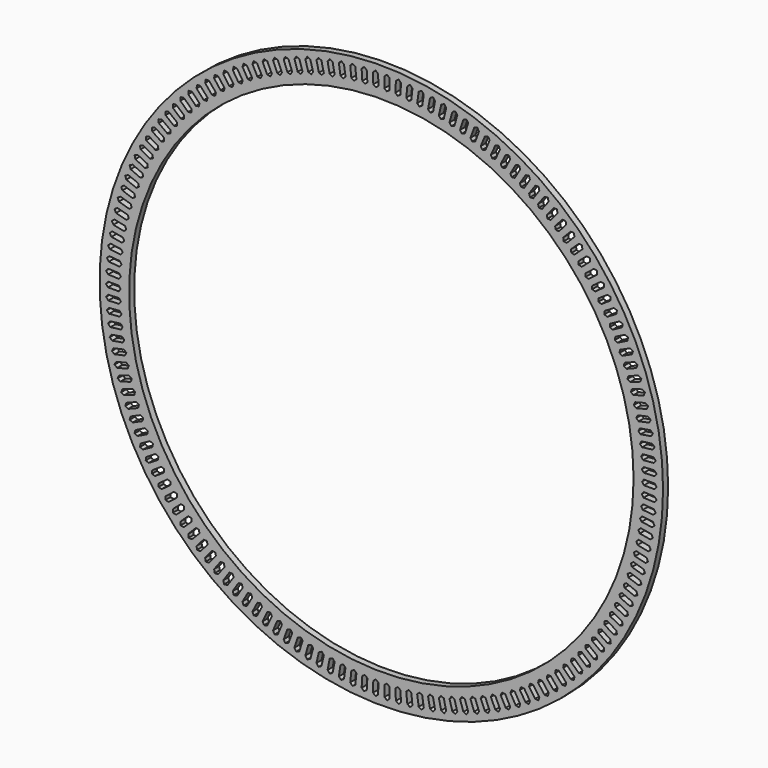
from build123d import *

# Parameters (mm, degrees)
F0_R     = 44.4451072214
F0_R_2   = 39.7909851914
F1_DEPTH = 1
F3_DEPTH = 1
F4_COUNT = 150
F6_SCALE = 2.61


with BuildPart() as f1:
    # F0 (on Front) → F1 (new body)
    with BuildSketch(Plane.XZ):
        Circle(F0_R)
        Circle(F0_R_2, mode=Mode.SUBTRACT)
    extrude(amount=-F1_DEPTH)


with BuildPart() as f3:
    # F2 (on Front) → F3 (new body)
    with BuildSketch(Plane.XZ):
        Polygon((-41.4202045649, 0.4029835982), (-43.1122351438, 0.4029835982), (-43.4538759291, 0), (-43.1122351438, -0.4029835982), (-41.4202045649, -0.4029835982), (-41.1230549216, 0), align=None)
    extrude(amount=-F3_DEPTH)


with BuildPart() as f4_1:
    # F4: instance of F3
    add(f3.part.rotate(Axis((0, 0, 0), (0, -1, 0)), 1 * 360 / F4_COUNT))


with BuildPart() as f4_2:
    # F4: instance of F3
    add(f3.part.rotate(Axis((0, 0, 0), (0, -1, 0)), 2 * 360 / F4_COUNT))


with BuildPart() as f4_3:
    # F4: instance of F3
    add(f3.part.rotate(Axis((0, 0, 0), (0, -1, 0)), 3 * 360 / F4_COUNT))


with BuildPart() as f4_4:
    # F4: instance of F3
    add(f3.part.rotate(Axis((0, 0, 0), (0, -1, 0)), 4 * 360 / F4_COUNT))


with BuildPart() as f4_5:
    # F4: instance of F3
    add(f3.part.rotate(Axis((0, 0, 0), (0, -1, 0)), 5 * 360 / F4_COUNT))


with BuildPart() as f4_6:
    # F4: instance of F3
    add(f3.part.rotate(Axis((0, 0, 0), (0, -1, 0)), 6 * 360 / F4_COUNT))


with BuildPart() as f4_7:
    # F4: instance of F3
    add(f3.part.rotate(Axis((0, 0, 0), (0, -1, 0)), 7 * 360 / F4_COUNT))


with BuildPart() as f4_8:
    # F4: instance of F3
    add(f3.part.rotate(Axis((0, 0, 0), (0, -1, 0)), 8 * 360 / F4_COUNT))


with BuildPart() as f4_9:
    # F4: instance of F3
    add(f3.part.rotate(Axis((0, 0, 0), (0, -1, 0)), 9 * 360 / F4_COUNT))


with BuildPart() as f4_10:
    # F4: instance of F3
    add(f3.part.rotate(Axis((0, 0, 0), (0, -1, 0)), 10 * 360 / F4_COUNT))


with BuildPart() as f4_11:
    # F4: instance of F3
    add(f3.part.rotate(Axis((0, 0, 0), (0, -1, 0)), 11 * 360 / F4_COUNT))


with BuildPart() as f4_12:
    # F4: instance of F3
    add(f3.part.rotate(Axis((0, 0, 0), (0, -1, 0)), 12 * 360 / F4_COUNT))


with BuildPart() as f4_13:
    # F4: instance of F3
    add(f3.part.rotate(Axis((0, 0, 0), (0, -1, 0)), 13 * 360 / F4_COUNT))


with BuildPart() as f4_14:
    # F4: instance of F3
    add(f3.part.rotate(Axis((0, 0, 0), (0, -1, 0)), 14 * 360 / F4_COUNT))


with BuildPart() as f4_15:
    # F4: instance of F3
    add(f3.part.rotate(Axis((0, 0, 0), (0, -1, 0)), 15 * 360 / F4_COUNT))


with BuildPart() as f4_16:
    # F4: instance of F3
    add(f3.part.rotate(Axis((0, 0, 0), (0, -1, 0)), 16 * 360 / F4_COUNT))


with BuildPart() as f4_17:
    # F4: instance of F3
    add(f3.part.rotate(Axis((0, 0, 0), (0, -1, 0)), 17 * 360 / F4_COUNT))


with BuildPart() as f4_18:
    # F4: instance of F3
    add(f3.part.rotate(Axis((0, 0, 0), (0, -1, 0)), 18 * 360 / F4_COUNT))


with BuildPart() as f4_19:
    # F4: instance of F3
    add(f3.part.rotate(Axis((0, 0, 0), (0, -1, 0)), 19 * 360 / F4_COUNT))


with BuildPart() as f4_20:
    # F4: instance of F3
    add(f3.part.rotate(Axis((0, 0, 0), (0, -1, 0)), 20 * 360 / F4_COUNT))


with BuildPart() as f4_21:
    # F4: instance of F3
    add(f3.part.rotate(Axis((0, 0, 0), (0, -1, 0)), 21 * 360 / F4_COUNT))


with BuildPart() as f4_22:
    # F4: instance of F3
    add(f3.part.rotate(Axis((0, 0, 0), (0, -1, 0)), 22 * 360 / F4_COUNT))


with BuildPart() as f4_23:
    # F4: instance of F3
    add(f3.part.rotate(Axis((0, 0, 0), (0, -1, 0)), 23 * 360 / F4_COUNT))


with BuildPart() as f4_24:
    # F4: instance of F3
    add(f3.part.rotate(Axis((0, 0, 0), (0, -1, 0)), 24 * 360 / F4_COUNT))


with BuildPart() as f4_25:
    # F4: instance of F3
    add(f3.part.rotate(Axis((0, 0, 0), (0, -1, 0)), 25 * 360 / F4_COUNT))


with BuildPart() as f4_26:
    # F4: instance of F3
    add(f3.part.rotate(Axis((0, 0, 0), (0, -1, 0)), 26 * 360 / F4_COUNT))


with BuildPart() as f4_27:
    # F4: instance of F3
    add(f3.part.rotate(Axis((0, 0, 0), (0, -1, 0)), 27 * 360 / F4_COUNT))


with BuildPart() as f4_28:
    # F4: instance of F3
    add(f3.part.rotate(Axis((0, 0, 0), (0, -1, 0)), 28 * 360 / F4_COUNT))


with BuildPart() as f4_29:
    # F4: instance of F3
    add(f3.part.rotate(Axis((0, 0, 0), (0, -1, 0)), 29 * 360 / F4_COUNT))


with BuildPart() as f4_30:
    # F4: instance of F3
    add(f3.part.rotate(Axis((0, 0, 0), (0, -1, 0)), 30 * 360 / F4_COUNT))


with BuildPart() as f4_31:
    # F4: instance of F3
    add(f3.part.rotate(Axis((0, 0, 0), (0, -1, 0)), 31 * 360 / F4_COUNT))


with BuildPart() as f4_32:
    # F4: instance of F3
    add(f3.part.rotate(Axis((0, 0, 0), (0, -1, 0)), 32 * 360 / F4_COUNT))


with BuildPart() as f4_33:
    # F4: instance of F3
    add(f3.part.rotate(Axis((0, 0, 0), (0, -1, 0)), 33 * 360 / F4_COUNT))


with BuildPart() as f4_34:
    # F4: instance of F3
    add(f3.part.rotate(Axis((0, 0, 0), (0, -1, 0)), 34 * 360 / F4_COUNT))


with BuildPart() as f4_35:
    # F4: instance of F3
    add(f3.part.rotate(Axis((0, 0, 0), (0, -1, 0)), 35 * 360 / F4_COUNT))


with BuildPart() as f4_36:
    # F4: instance of F3
    add(f3.part.rotate(Axis((0, 0, 0), (0, -1, 0)), 36 * 360 / F4_COUNT))


with BuildPart() as f4_37:
    # F4: instance of F3
    add(f3.part.rotate(Axis((0, 0, 0), (0, -1, 0)), 37 * 360 / F4_COUNT))


with BuildPart() as f4_38:
    # F4: instance of F3
    add(f3.part.rotate(Axis((0, 0, 0), (0, -1, 0)), 38 * 360 / F4_COUNT))


with BuildPart() as f4_39:
    # F4: instance of F3
    add(f3.part.rotate(Axis((0, 0, 0), (0, -1, 0)), 39 * 360 / F4_COUNT))


with BuildPart() as f4_40:
    # F4: instance of F3
    add(f3.part.rotate(Axis((0, 0, 0), (0, -1, 0)), 40 * 360 / F4_COUNT))


with BuildPart() as f4_41:
    # F4: instance of F3
    add(f3.part.rotate(Axis((0, 0, 0), (0, -1, 0)), 41 * 360 / F4_COUNT))


with BuildPart() as f4_42:
    # F4: instance of F3
    add(f3.part.rotate(Axis((0, 0, 0), (0, -1, 0)), 42 * 360 / F4_COUNT))


with BuildPart() as f4_43:
    # F4: instance of F3
    add(f3.part.rotate(Axis((0, 0, 0), (0, -1, 0)), 43 * 360 / F4_COUNT))


with BuildPart() as f4_44:
    # F4: instance of F3
    add(f3.part.rotate(Axis((0, 0, 0), (0, -1, 0)), 44 * 360 / F4_COUNT))


with BuildPart() as f4_45:
    # F4: instance of F3
    add(f3.part.rotate(Axis((0, 0, 0), (0, -1, 0)), 45 * 360 / F4_COUNT))


with BuildPart() as f4_46:
    # F4: instance of F3
    add(f3.part.rotate(Axis((0, 0, 0), (0, -1, 0)), 46 * 360 / F4_COUNT))


with BuildPart() as f4_47:
    # F4: instance of F3
    add(f3.part.rotate(Axis((0, 0, 0), (0, -1, 0)), 47 * 360 / F4_COUNT))


with BuildPart() as f4_48:
    # F4: instance of F3
    add(f3.part.rotate(Axis((0, 0, 0), (0, -1, 0)), 48 * 360 / F4_COUNT))


with BuildPart() as f4_49:
    # F4: instance of F3
    add(f3.part.rotate(Axis((0, 0, 0), (0, -1, 0)), 49 * 360 / F4_COUNT))


with BuildPart() as f4_50:
    # F4: instance of F3
    add(f3.part.rotate(Axis((0, 0, 0), (0, -1, 0)), 50 * 360 / F4_COUNT))


with BuildPart() as f4_51:
    # F4: instance of F3
    add(f3.part.rotate(Axis((0, 0, 0), (0, -1, 0)), 51 * 360 / F4_COUNT))


with BuildPart() as f4_52:
    # F4: instance of F3
    add(f3.part.rotate(Axis((0, 0, 0), (0, -1, 0)), 52 * 360 / F4_COUNT))


with BuildPart() as f4_53:
    # F4: instance of F3
    add(f3.part.rotate(Axis((0, 0, 0), (0, -1, 0)), 53 * 360 / F4_COUNT))


with BuildPart() as f4_54:
    # F4: instance of F3
    add(f3.part.rotate(Axis((0, 0, 0), (0, -1, 0)), 54 * 360 / F4_COUNT))


with BuildPart() as f4_55:
    # F4: instance of F3
    add(f3.part.rotate(Axis((0, 0, 0), (0, -1, 0)), 55 * 360 / F4_COUNT))


with BuildPart() as f4_56:
    # F4: instance of F3
    add(f3.part.rotate(Axis((0, 0, 0), (0, -1, 0)), 56 * 360 / F4_COUNT))


with BuildPart() as f4_57:
    # F4: instance of F3
    add(f3.part.rotate(Axis((0, 0, 0), (0, -1, 0)), 57 * 360 / F4_COUNT))


with BuildPart() as f4_58:
    # F4: instance of F3
    add(f3.part.rotate(Axis((0, 0, 0), (0, -1, 0)), 58 * 360 / F4_COUNT))


with BuildPart() as f4_59:
    # F4: instance of F3
    add(f3.part.rotate(Axis((0, 0, 0), (0, -1, 0)), 59 * 360 / F4_COUNT))


with BuildPart() as f4_60:
    # F4: instance of F3
    add(f3.part.rotate(Axis((0, 0, 0), (0, -1, 0)), 60 * 360 / F4_COUNT))


with BuildPart() as f4_61:
    # F4: instance of F3
    add(f3.part.rotate(Axis((0, 0, 0), (0, -1, 0)), 61 * 360 / F4_COUNT))


with BuildPart() as f4_62:
    # F4: instance of F3
    add(f3.part.rotate(Axis((0, 0, 0), (0, -1, 0)), 62 * 360 / F4_COUNT))


with BuildPart() as f4_63:
    # F4: instance of F3
    add(f3.part.rotate(Axis((0, 0, 0), (0, -1, 0)), 63 * 360 / F4_COUNT))


with BuildPart() as f4_64:
    # F4: instance of F3
    add(f3.part.rotate(Axis((0, 0, 0), (0, -1, 0)), 64 * 360 / F4_COUNT))


with BuildPart() as f4_65:
    # F4: instance of F3
    add(f3.part.rotate(Axis((0, 0, 0), (0, -1, 0)), 65 * 360 / F4_COUNT))


with BuildPart() as f4_66:
    # F4: instance of F3
    add(f3.part.rotate(Axis((0, 0, 0), (0, -1, 0)), 66 * 360 / F4_COUNT))


with BuildPart() as f4_67:
    # F4: instance of F3
    add(f3.part.rotate(Axis((0, 0, 0), (0, -1, 0)), 67 * 360 / F4_COUNT))


with BuildPart() as f4_68:
    # F4: instance of F3
    add(f3.part.rotate(Axis((0, 0, 0), (0, -1, 0)), 68 * 360 / F4_COUNT))


with BuildPart() as f4_69:
    # F4: instance of F3
    add(f3.part.rotate(Axis((0, 0, 0), (0, -1, 0)), 69 * 360 / F4_COUNT))


with BuildPart() as f4_70:
    # F4: instance of F3
    add(f3.part.rotate(Axis((0, 0, 0), (0, -1, 0)), 70 * 360 / F4_COUNT))


with BuildPart() as f4_71:
    # F4: instance of F3
    add(f3.part.rotate(Axis((0, 0, 0), (0, -1, 0)), 71 * 360 / F4_COUNT))


with BuildPart() as f4_72:
    # F4: instance of F3
    add(f3.part.rotate(Axis((0, 0, 0), (0, -1, 0)), 72 * 360 / F4_COUNT))


with BuildPart() as f4_73:
    # F4: instance of F3
    add(f3.part.rotate(Axis((0, 0, 0), (0, -1, 0)), 73 * 360 / F4_COUNT))


with BuildPart() as f4_74:
    # F4: instance of F3
    add(f3.part.rotate(Axis((0, 0, 0), (0, -1, 0)), 74 * 360 / F4_COUNT))


with BuildPart() as f4_75:
    # F4: instance of F3
    add(f3.part.rotate(Axis((0, 0, 0), (0, -1, 0)), 75 * 360 / F4_COUNT))


with BuildPart() as f4_76:
    # F4: instance of F3
    add(f3.part.rotate(Axis((0, 0, 0), (0, -1, 0)), 76 * 360 / F4_COUNT))


with BuildPart() as f4_77:
    # F4: instance of F3
    add(f3.part.rotate(Axis((0, 0, 0), (0, -1, 0)), 77 * 360 / F4_COUNT))


with BuildPart() as f4_78:
    # F4: instance of F3
    add(f3.part.rotate(Axis((0, 0, 0), (0, -1, 0)), 78 * 360 / F4_COUNT))


with BuildPart() as f4_79:
    # F4: instance of F3
    add(f3.part.rotate(Axis((0, 0, 0), (0, -1, 0)), 79 * 360 / F4_COUNT))


with BuildPart() as f4_80:
    # F4: instance of F3
    add(f3.part.rotate(Axis((0, 0, 0), (0, -1, 0)), 80 * 360 / F4_COUNT))


with BuildPart() as f4_81:
    # F4: instance of F3
    add(f3.part.rotate(Axis((0, 0, 0), (0, -1, 0)), 81 * 360 / F4_COUNT))


with BuildPart() as f4_82:
    # F4: instance of F3
    add(f3.part.rotate(Axis((0, 0, 0), (0, -1, 0)), 82 * 360 / F4_COUNT))


with BuildPart() as f4_83:
    # F4: instance of F3
    add(f3.part.rotate(Axis((0, 0, 0), (0, -1, 0)), 83 * 360 / F4_COUNT))


with BuildPart() as f4_84:
    # F4: instance of F3
    add(f3.part.rotate(Axis((0, 0, 0), (0, -1, 0)), 84 * 360 / F4_COUNT))


with BuildPart() as f4_85:
    # F4: instance of F3
    add(f3.part.rotate(Axis((0, 0, 0), (0, -1, 0)), 85 * 360 / F4_COUNT))


with BuildPart() as f4_86:
    # F4: instance of F3
    add(f3.part.rotate(Axis((0, 0, 0), (0, -1, 0)), 86 * 360 / F4_COUNT))


with BuildPart() as f4_87:
    # F4: instance of F3
    add(f3.part.rotate(Axis((0, 0, 0), (0, -1, 0)), 87 * 360 / F4_COUNT))


with BuildPart() as f4_88:
    # F4: instance of F3
    add(f3.part.rotate(Axis((0, 0, 0), (0, -1, 0)), 88 * 360 / F4_COUNT))


with BuildPart() as f4_89:
    # F4: instance of F3
    add(f3.part.rotate(Axis((0, 0, 0), (0, -1, 0)), 89 * 360 / F4_COUNT))


with BuildPart() as f4_90:
    # F4: instance of F3
    add(f3.part.rotate(Axis((0, 0, 0), (0, -1, 0)), 90 * 360 / F4_COUNT))


with BuildPart() as f4_91:
    # F4: instance of F3
    add(f3.part.rotate(Axis((0, 0, 0), (0, -1, 0)), 91 * 360 / F4_COUNT))


with BuildPart() as f4_92:
    # F4: instance of F3
    add(f3.part.rotate(Axis((0, 0, 0), (0, -1, 0)), 92 * 360 / F4_COUNT))


with BuildPart() as f4_93:
    # F4: instance of F3
    add(f3.part.rotate(Axis((0, 0, 0), (0, -1, 0)), 93 * 360 / F4_COUNT))


with BuildPart() as f4_94:
    # F4: instance of F3
    add(f3.part.rotate(Axis((0, 0, 0), (0, -1, 0)), 94 * 360 / F4_COUNT))


with BuildPart() as f4_95:
    # F4: instance of F3
    add(f3.part.rotate(Axis((0, 0, 0), (0, -1, 0)), 95 * 360 / F4_COUNT))


with BuildPart() as f4_96:
    # F4: instance of F3
    add(f3.part.rotate(Axis((0, 0, 0), (0, -1, 0)), 96 * 360 / F4_COUNT))


with BuildPart() as f4_97:
    # F4: instance of F3
    add(f3.part.rotate(Axis((0, 0, 0), (0, -1, 0)), 97 * 360 / F4_COUNT))


with BuildPart() as f4_98:
    # F4: instance of F3
    add(f3.part.rotate(Axis((0, 0, 0), (0, -1, 0)), 98 * 360 / F4_COUNT))


with BuildPart() as f4_99:
    # F4: instance of F3
    add(f3.part.rotate(Axis((0, 0, 0), (0, -1, 0)), 99 * 360 / F4_COUNT))


with BuildPart() as f4_100:
    # F4: instance of F3
    add(f3.part.rotate(Axis((0, 0, 0), (0, -1, 0)), 100 * 360 / F4_COUNT))


with BuildPart() as f4_101:
    # F4: instance of F3
    add(f3.part.rotate(Axis((0, 0, 0), (0, -1, 0)), 101 * 360 / F4_COUNT))


with BuildPart() as f4_102:
    # F4: instance of F3
    add(f3.part.rotate(Axis((0, 0, 0), (0, -1, 0)), 102 * 360 / F4_COUNT))


with BuildPart() as f4_103:
    # F4: instance of F3
    add(f3.part.rotate(Axis((0, 0, 0), (0, -1, 0)), 103 * 360 / F4_COUNT))


with BuildPart() as f4_104:
    # F4: instance of F3
    add(f3.part.rotate(Axis((0, 0, 0), (0, -1, 0)), 104 * 360 / F4_COUNT))


with BuildPart() as f4_105:
    # F4: instance of F3
    add(f3.part.rotate(Axis((0, 0, 0), (0, -1, 0)), 105 * 360 / F4_COUNT))


with BuildPart() as f4_106:
    # F4: instance of F3
    add(f3.part.rotate(Axis((0, 0, 0), (0, -1, 0)), 106 * 360 / F4_COUNT))


with BuildPart() as f4_107:
    # F4: instance of F3
    add(f3.part.rotate(Axis((0, 0, 0), (0, -1, 0)), 107 * 360 / F4_COUNT))


with BuildPart() as f4_108:
    # F4: instance of F3
    add(f3.part.rotate(Axis((0, 0, 0), (0, -1, 0)), 108 * 360 / F4_COUNT))


with BuildPart() as f4_109:
    # F4: instance of F3
    add(f3.part.rotate(Axis((0, 0, 0), (0, -1, 0)), 109 * 360 / F4_COUNT))


with BuildPart() as f4_110:
    # F4: instance of F3
    add(f3.part.rotate(Axis((0, 0, 0), (0, -1, 0)), 110 * 360 / F4_COUNT))


with BuildPart() as f4_111:
    # F4: instance of F3
    add(f3.part.rotate(Axis((0, 0, 0), (0, -1, 0)), 111 * 360 / F4_COUNT))


with BuildPart() as f4_112:
    # F4: instance of F3
    add(f3.part.rotate(Axis((0, 0, 0), (0, -1, 0)), 112 * 360 / F4_COUNT))


with BuildPart() as f4_113:
    # F4: instance of F3
    add(f3.part.rotate(Axis((0, 0, 0), (0, -1, 0)), 113 * 360 / F4_COUNT))


with BuildPart() as f4_114:
    # F4: instance of F3
    add(f3.part.rotate(Axis((0, 0, 0), (0, -1, 0)), 114 * 360 / F4_COUNT))


with BuildPart() as f4_115:
    # F4: instance of F3
    add(f3.part.rotate(Axis((0, 0, 0), (0, -1, 0)), 115 * 360 / F4_COUNT))


with BuildPart() as f4_116:
    # F4: instance of F3
    add(f3.part.rotate(Axis((0, 0, 0), (0, -1, 0)), 116 * 360 / F4_COUNT))


with BuildPart() as f4_117:
    # F4: instance of F3
    add(f3.part.rotate(Axis((0, 0, 0), (0, -1, 0)), 117 * 360 / F4_COUNT))


with BuildPart() as f4_118:
    # F4: instance of F3
    add(f3.part.rotate(Axis((0, 0, 0), (0, -1, 0)), 118 * 360 / F4_COUNT))


with BuildPart() as f4_119:
    # F4: instance of F3
    add(f3.part.rotate(Axis((0, 0, 0), (0, -1, 0)), 119 * 360 / F4_COUNT))


with BuildPart() as f4_120:
    # F4: instance of F3
    add(f3.part.rotate(Axis((0, 0, 0), (0, -1, 0)), 120 * 360 / F4_COUNT))


with BuildPart() as f4_121:
    # F4: instance of F3
    add(f3.part.rotate(Axis((0, 0, 0), (0, -1, 0)), 121 * 360 / F4_COUNT))


with BuildPart() as f4_122:
    # F4: instance of F3
    add(f3.part.rotate(Axis((0, 0, 0), (0, -1, 0)), 122 * 360 / F4_COUNT))


with BuildPart() as f4_123:
    # F4: instance of F3
    add(f3.part.rotate(Axis((0, 0, 0), (0, -1, 0)), 123 * 360 / F4_COUNT))


with BuildPart() as f4_124:
    # F4: instance of F3
    add(f3.part.rotate(Axis((0, 0, 0), (0, -1, 0)), 124 * 360 / F4_COUNT))


with BuildPart() as f4_125:
    # F4: instance of F3
    add(f3.part.rotate(Axis((0, 0, 0), (0, -1, 0)), 125 * 360 / F4_COUNT))


with BuildPart() as f4_126:
    # F4: instance of F3
    add(f3.part.rotate(Axis((0, 0, 0), (0, -1, 0)), 126 * 360 / F4_COUNT))


with BuildPart() as f4_127:
    # F4: instance of F3
    add(f3.part.rotate(Axis((0, 0, 0), (0, -1, 0)), 127 * 360 / F4_COUNT))


with BuildPart() as f4_128:
    # F4: instance of F3
    add(f3.part.rotate(Axis((0, 0, 0), (0, -1, 0)), 128 * 360 / F4_COUNT))


with BuildPart() as f4_129:
    # F4: instance of F3
    add(f3.part.rotate(Axis((0, 0, 0), (0, -1, 0)), 129 * 360 / F4_COUNT))


with BuildPart() as f4_130:
    # F4: instance of F3
    add(f3.part.rotate(Axis((0, 0, 0), (0, -1, 0)), 130 * 360 / F4_COUNT))


with BuildPart() as f4_131:
    # F4: instance of F3
    add(f3.part.rotate(Axis((0, 0, 0), (0, -1, 0)), 131 * 360 / F4_COUNT))


with BuildPart() as f4_132:
    # F4: instance of F3
    add(f3.part.rotate(Axis((0, 0, 0), (0, -1, 0)), 132 * 360 / F4_COUNT))


with BuildPart() as f4_133:
    # F4: instance of F3
    add(f3.part.rotate(Axis((0, 0, 0), (0, -1, 0)), 133 * 360 / F4_COUNT))


with BuildPart() as f4_134:
    # F4: instance of F3
    add(f3.part.rotate(Axis((0, 0, 0), (0, -1, 0)), 134 * 360 / F4_COUNT))


with BuildPart() as f4_135:
    # F4: instance of F3
    add(f3.part.rotate(Axis((0, 0, 0), (0, -1, 0)), 135 * 360 / F4_COUNT))


with BuildPart() as f4_136:
    # F4: instance of F3
    add(f3.part.rotate(Axis((0, 0, 0), (0, -1, 0)), 136 * 360 / F4_COUNT))


with BuildPart() as f4_137:
    # F4: instance of F3
    add(f3.part.rotate(Axis((0, 0, 0), (0, -1, 0)), 137 * 360 / F4_COUNT))


with BuildPart() as f4_138:
    # F4: instance of F3
    add(f3.part.rotate(Axis((0, 0, 0), (0, -1, 0)), 138 * 360 / F4_COUNT))


with BuildPart() as f4_139:
    # F4: instance of F3
    add(f3.part.rotate(Axis((0, 0, 0), (0, -1, 0)), 139 * 360 / F4_COUNT))


with BuildPart() as f4_140:
    # F4: instance of F3
    add(f3.part.rotate(Axis((0, 0, 0), (0, -1, 0)), 140 * 360 / F4_COUNT))


with BuildPart() as f4_141:
    # F4: instance of F3
    add(f3.part.rotate(Axis((0, 0, 0), (0, -1, 0)), 141 * 360 / F4_COUNT))


with BuildPart() as f4_142:
    # F4: instance of F3
    add(f3.part.rotate(Axis((0, 0, 0), (0, -1, 0)), 142 * 360 / F4_COUNT))


with BuildPart() as f4_143:
    # F4: instance of F3
    add(f3.part.rotate(Axis((0, 0, 0), (0, -1, 0)), 143 * 360 / F4_COUNT))


with BuildPart() as f4_144:
    # F4: instance of F3
    add(f3.part.rotate(Axis((0, 0, 0), (0, -1, 0)), 144 * 360 / F4_COUNT))


with BuildPart() as f4_145:
    # F4: instance of F3
    add(f3.part.rotate(Axis((0, 0, 0), (0, -1, 0)), 145 * 360 / F4_COUNT))


with BuildPart() as f4_146:
    # F4: instance of F3
    add(f3.part.rotate(Axis((0, 0, 0), (0, -1, 0)), 146 * 360 / F4_COUNT))


with BuildPart() as f4_147:
    # F4: instance of F3
    add(f3.part.rotate(Axis((0, 0, 0), (0, -1, 0)), 147 * 360 / F4_COUNT))


with BuildPart() as f4_148:
    # F4: instance of F3
    add(f3.part.rotate(Axis((0, 0, 0), (0, -1, 0)), 148 * 360 / F4_COUNT))


with BuildPart() as f4_149:
    # F4: instance of F3
    add(f3.part.rotate(Axis((0, 0, 0), (0, -1, 0)), 149 * 360 / F4_COUNT))


with BuildPart() as f1_1:
    add(f1.part)

    # F5: cut F4_5, F4_6, F4_4, F4_23, F4_21, F4_24, F4_22, F4_20, F4_19, F4_18, F4_17, F4_16, F4_15, F4_14, F4_13, F4_12, F4_11, F4_10, F4_9, F4_8, F4_7, F4_1, F4_3, F4_2, F3, F4_149, F4_148, F4_147, F4_25, F4_26, F4_27, F4_28, F4_29, F4_30, F4_31, F4_32, F4_33, F4_34, F4_35, F4_36, F4_37, F4_38, F4_39, F4_40, F4_41, F4_42, F4_43, F4_44, F4_45, F4_46, F4_47, F4_48, F4_49, F4_50, F4_51, F4_52, F4_53, F4_54, F4_55, F4_56, F4_57, F4_58, F4_59, F4_60, F4_61, F4_62, F4_63, F4_64, F4_65, F4_66, F4_67, F4_68, F4_69, F4_70, F4_71, F4_72, F4_73, F4_74, F4_75, F4_76, F4_77, F4_78, F4_79, F4_80, F4_81, F4_82, F4_83, F4_84, F4_85, F4_86, F4_87, F4_88, F4_89, F4_90, F4_91, F4_92, F4_93, F4_94, F4_95, F4_96, F4_97, F4_98, F4_99, F4_100, F4_101, F4_102, F4_103, F4_104, F4_105, F4_106, F4_107, F4_108, F4_109, F4_110, F4_111, F4_112, F4_113, F4_114, F4_115, F4_116, F4_117, F4_118, F4_119, F4_120, F4_121, F4_122, F4_123, F4_124, F4_125, F4_126, F4_127, F4_128, F4_129, F4_130, F4_131, F4_132, F4_133, F4_134, F4_135, F4_136, F4_137, F4_138, F4_139, F4_140, F4_141, F4_142, F4_143, F4_144, F4_145, F4_146
    add(f4_5.part, mode=Mode.SUBTRACT)
    add(f4_6.part, mode=Mode.SUBTRACT)
    add(f4_4.part, mode=Mode.SUBTRACT)
    add(f4_23.part, mode=Mode.SUBTRACT)
    add(f4_21.part, mode=Mode.SUBTRACT)
    add(f4_24.part, mode=Mode.SUBTRACT)
    add(f4_22.part, mode=Mode.SUBTRACT)
    add(f4_20.part, mode=Mode.SUBTRACT)
    add(f4_19.part, mode=Mode.SUBTRACT)
    add(f4_18.part, mode=Mode.SUBTRACT)
    add(f4_17.part, mode=Mode.SUBTRACT)
    add(f4_16.part, mode=Mode.SUBTRACT)
    add(f4_15.part, mode=Mode.SUBTRACT)
    add(f4_14.part, mode=Mode.SUBTRACT)
    add(f4_13.part, mode=Mode.SUBTRACT)
    add(f4_12.part, mode=Mode.SUBTRACT)
    add(f4_11.part, mode=Mode.SUBTRACT)
    add(f4_10.part, mode=Mode.SUBTRACT)
    add(f4_9.part, mode=Mode.SUBTRACT)
    add(f4_8.part, mode=Mode.SUBTRACT)
    add(f4_7.part, mode=Mode.SUBTRACT)
    add(f4_1.part, mode=Mode.SUBTRACT)
    add(f4_3.part, mode=Mode.SUBTRACT)
    add(f4_2.part, mode=Mode.SUBTRACT)
    add(f3.part, mode=Mode.SUBTRACT)
    add(f4_149.part, mode=Mode.SUBTRACT)
    add(f4_148.part, mode=Mode.SUBTRACT)
    add(f4_147.part, mode=Mode.SUBTRACT)
    add(f4_25.part, mode=Mode.SUBTRACT)
    add(f4_26.part, mode=Mode.SUBTRACT)
    add(f4_27.part, mode=Mode.SUBTRACT)
    add(f4_28.part, mode=Mode.SUBTRACT)
    add(f4_29.part, mode=Mode.SUBTRACT)
    add(f4_30.part, mode=Mode.SUBTRACT)
    add(f4_31.part, mode=Mode.SUBTRACT)
    add(f4_32.part, mode=Mode.SUBTRACT)
    add(f4_33.part, mode=Mode.SUBTRACT)
    add(f4_34.part, mode=Mode.SUBTRACT)
    add(f4_35.part, mode=Mode.SUBTRACT)
    add(f4_36.part, mode=Mode.SUBTRACT)
    add(f4_37.part, mode=Mode.SUBTRACT)
    add(f4_38.part, mode=Mode.SUBTRACT)
    add(f4_39.part, mode=Mode.SUBTRACT)
    add(f4_40.part, mode=Mode.SUBTRACT)
    add(f4_41.part, mode=Mode.SUBTRACT)
    add(f4_42.part, mode=Mode.SUBTRACT)
    add(f4_43.part, mode=Mode.SUBTRACT)
    add(f4_44.part, mode=Mode.SUBTRACT)
    add(f4_45.part, mode=Mode.SUBTRACT)
    add(f4_46.part, mode=Mode.SUBTRACT)
    add(f4_47.part, mode=Mode.SUBTRACT)
    add(f4_48.part, mode=Mode.SUBTRACT)
    add(f4_49.part, mode=Mode.SUBTRACT)
    add(f4_50.part, mode=Mode.SUBTRACT)
    add(f4_51.part, mode=Mode.SUBTRACT)
    add(f4_52.part, mode=Mode.SUBTRACT)
    add(f4_53.part, mode=Mode.SUBTRACT)
    add(f4_54.part, mode=Mode.SUBTRACT)
    add(f4_55.part, mode=Mode.SUBTRACT)
    add(f4_56.part, mode=Mode.SUBTRACT)
    add(f4_57.part, mode=Mode.SUBTRACT)
    add(f4_58.part, mode=Mode.SUBTRACT)
    add(f4_59.part, mode=Mode.SUBTRACT)
    add(f4_60.part, mode=Mode.SUBTRACT)
    add(f4_61.part, mode=Mode.SUBTRACT)
    add(f4_62.part, mode=Mode.SUBTRACT)
    add(f4_63.part, mode=Mode.SUBTRACT)
    add(f4_64.part, mode=Mode.SUBTRACT)
    add(f4_65.part, mode=Mode.SUBTRACT)
    add(f4_66.part, mode=Mode.SUBTRACT)
    add(f4_67.part, mode=Mode.SUBTRACT)
    add(f4_68.part, mode=Mode.SUBTRACT)
    add(f4_69.part, mode=Mode.SUBTRACT)
    add(f4_70.part, mode=Mode.SUBTRACT)
    add(f4_71.part, mode=Mode.SUBTRACT)
    add(f4_72.part, mode=Mode.SUBTRACT)
    add(f4_73.part, mode=Mode.SUBTRACT)
    add(f4_74.part, mode=Mode.SUBTRACT)
    add(f4_75.part, mode=Mode.SUBTRACT)
    add(f4_76.part, mode=Mode.SUBTRACT)
    add(f4_77.part, mode=Mode.SUBTRACT)
    add(f4_78.part, mode=Mode.SUBTRACT)
    add(f4_79.part, mode=Mode.SUBTRACT)
    add(f4_80.part, mode=Mode.SUBTRACT)
    add(f4_81.part, mode=Mode.SUBTRACT)
    add(f4_82.part, mode=Mode.SUBTRACT)
    add(f4_83.part, mode=Mode.SUBTRACT)
    add(f4_84.part, mode=Mode.SUBTRACT)
    add(f4_85.part, mode=Mode.SUBTRACT)
    add(f4_86.part, mode=Mode.SUBTRACT)
    add(f4_87.part, mode=Mode.SUBTRACT)
    add(f4_88.part, mode=Mode.SUBTRACT)
    add(f4_89.part, mode=Mode.SUBTRACT)
    add(f4_90.part, mode=Mode.SUBTRACT)
    add(f4_91.part, mode=Mode.SUBTRACT)
    add(f4_92.part, mode=Mode.SUBTRACT)
    add(f4_93.part, mode=Mode.SUBTRACT)
    add(f4_94.part, mode=Mode.SUBTRACT)
    add(f4_95.part, mode=Mode.SUBTRACT)
    add(f4_96.part, mode=Mode.SUBTRACT)
    add(f4_97.part, mode=Mode.SUBTRACT)
    add(f4_98.part, mode=Mode.SUBTRACT)
    add(f4_99.part, mode=Mode.SUBTRACT)
    add(f4_100.part, mode=Mode.SUBTRACT)
    add(f4_101.part, mode=Mode.SUBTRACT)
    add(f4_102.part, mode=Mode.SUBTRACT)
    add(f4_103.part, mode=Mode.SUBTRACT)
    add(f4_104.part, mode=Mode.SUBTRACT)
    add(f4_105.part, mode=Mode.SUBTRACT)
    add(f4_106.part, mode=Mode.SUBTRACT)
    add(f4_107.part, mode=Mode.SUBTRACT)
    add(f4_108.part, mode=Mode.SUBTRACT)
    add(f4_109.part, mode=Mode.SUBTRACT)
    add(f4_110.part, mode=Mode.SUBTRACT)
    add(f4_111.part, mode=Mode.SUBTRACT)
    add(f4_112.part, mode=Mode.SUBTRACT)
    add(f4_113.part, mode=Mode.SUBTRACT)
    add(f4_114.part, mode=Mode.SUBTRACT)
    add(f4_115.part, mode=Mode.SUBTRACT)
    add(f4_116.part, mode=Mode.SUBTRACT)
    add(f4_117.part, mode=Mode.SUBTRACT)
    add(f4_118.part, mode=Mode.SUBTRACT)
    add(f4_119.part, mode=Mode.SUBTRACT)
    add(f4_120.part, mode=Mode.SUBTRACT)
    add(f4_121.part, mode=Mode.SUBTRACT)
    add(f4_122.part, mode=Mode.SUBTRACT)
    add(f4_123.part, mode=Mode.SUBTRACT)
    add(f4_124.part, mode=Mode.SUBTRACT)
    add(f4_125.part, mode=Mode.SUBTRACT)
    add(f4_126.part, mode=Mode.SUBTRACT)
    add(f4_127.part, mode=Mode.SUBTRACT)
    add(f4_128.part, mode=Mode.SUBTRACT)
    add(f4_129.part, mode=Mode.SUBTRACT)
    add(f4_130.part, mode=Mode.SUBTRACT)
    add(f4_131.part, mode=Mode.SUBTRACT)
    add(f4_132.part, mode=Mode.SUBTRACT)
    add(f4_133.part, mode=Mode.SUBTRACT)
    add(f4_134.part, mode=Mode.SUBTRACT)
    add(f4_135.part, mode=Mode.SUBTRACT)
    add(f4_136.part, mode=Mode.SUBTRACT)
    add(f4_137.part, mode=Mode.SUBTRACT)
    add(f4_138.part, mode=Mode.SUBTRACT)
    add(f4_139.part, mode=Mode.SUBTRACT)
    add(f4_140.part, mode=Mode.SUBTRACT)
    add(f4_141.part, mode=Mode.SUBTRACT)
    add(f4_142.part, mode=Mode.SUBTRACT)
    add(f4_143.part, mode=Mode.SUBTRACT)
    add(f4_144.part, mode=Mode.SUBTRACT)
    add(f4_145.part, mode=Mode.SUBTRACT)
    add(f4_146.part, mode=Mode.SUBTRACT)


with BuildPart() as f1_2:
    # F6: moved
    add(f1_1.part.scale(F6_SCALE))


solid = f1_2.part
